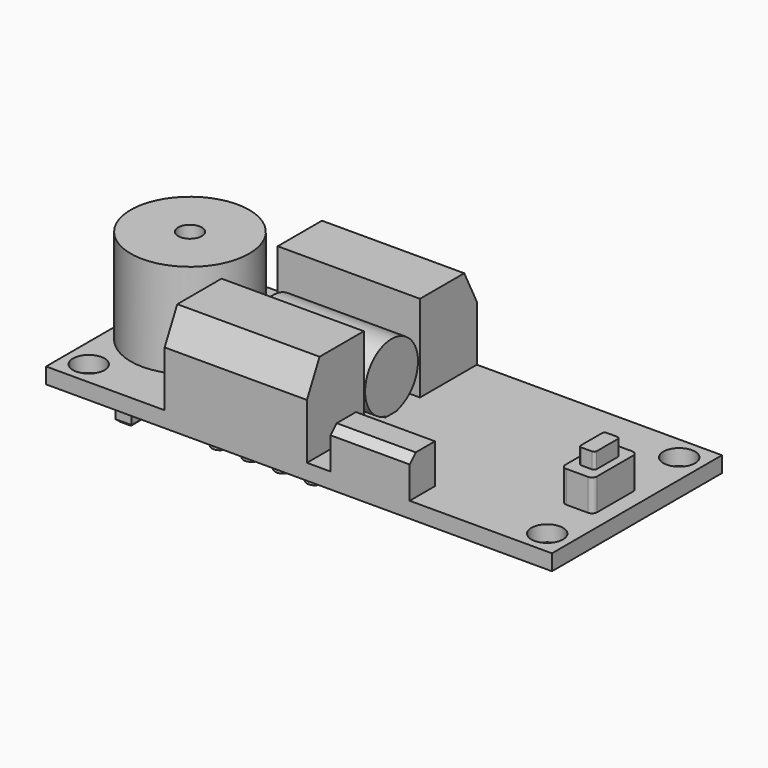
from build123d import *

# Parameters (mm, degrees)
F0_W      = 50.8
F0_H      = 21.336
F1_DEPTH  = 1.5875
F2_R      = 1.5875
F3_DEPTH  = 3.175
F5_DEPTH  = 2.38125
F6_W      = 1.5875
F6_H      = 2.38125
F6_W_2    = 5.55625
F6_H_2    = 3.96875
F6_W_3    = 2.38125
F6_H_3    = 3.175
F6_W_4    = 6.35
F6_H_4    = 4.7625
F7_DEPTH  = 1.5875
F8_SIZE   = 0.254
F9_W      = 5.55625
F9_H      = 7.14375
F10_DEPTH = 2.38125
F11_SIZE  = 0.762
F12_SIZE  = 0.254
F13_R     = 5.953125
F14_DEPTH = 9.525
F15_R     = 1.190625
F16_DEPTH = 3.175
F17_W     = 14.2875
F17_H     = 7.14375
F18_DEPTH = 8.73125
F20_DEPTH = 15.24
F22_DEPTH = 11.90625
F23_W     = 3.175
F23_H     = 5.55625
F24_DEPTH = 3.175
F25_W     = 1.5875
F25_H     = 3.175
F26_DEPTH = 1.5875
F27_R     = 0.254
F28_R     = 0.508
F29_W     = 7.9375
F29_H     = 3.175
F30_DEPTH = 3.96875
F31_SIZE  = 0.762


# Not quite as in the source:
# - a length typed as a fraction of an inch, garbled in the dataset ("3 / 203.2 mm" for 3/8 in), is restored


with BuildPart() as f1:
    # F0 (on Top) → F1 (new body)
    with BuildSketch(Plane.XY):
        with Locations((2.7589667588, 1.2681204271)):
            Rectangle(F0_W, F0_H)
    extrude(amount=F1_DEPTH)

    # F2 (on face) → F3 (cut)
    with BuildSketch(Plane.XY.offset(1.5875)):
        with Locations((25.7777167588, -7.0186295729)):
            Circle(F2_R)
        with Locations((25.7777167588, 9.5548704271)):
            Circle(F2_R)
        with Locations((-20.2597832412, 9.5548704271)):
            Circle(F2_R)
        with Locations((-20.2597832412, -7.0186295729)):
            Circle(F2_R)
    extrude(amount=-F3_DEPTH, mode=Mode.SUBTRACT)

    # F4 (on face) → F5 (join)
    with BuildSketch(Plane(origin=(0, 0, 0), x_dir=(1, 0, 0), z_dir=(0, 0, -1))):
        with BuildLine():
            ThreePointArc((-5.1785332412, 6.2248795729), (-5.9722832412, 5.4311295706), (-5.1785332365, 4.6373795729))
            ThreePointArc((-5.1785332365, 4.6373795729), (-4.6172672319, 4.869863567), (-4.3847832412, 5.4311295729))
            ThreePointArc((-4.3847832412, 5.4311295729), (-4.6172672336, 5.9923955805), (-5.1785332412, 6.2248795729))
        make_face()
        with BuildLine():
            ThreePointArc((-2.0035332412, 6.2248795729), (-2.7972832412, 5.4311295729), (-2.0035332412, 4.6373795729))
            ThreePointArc((-2.0035332412, 4.6373795729), (-1.4422672336, 4.8698635653), (-1.2097832412, 5.4311295729))
            ThreePointArc((-1.2097832412, 5.4311295729), (-1.4422672336, 5.9923955805), (-2.0035332412, 6.2248795729))
        make_face()
        with BuildLine():
            ThreePointArc((1.1714667642, 6.2248795729), (0.3777167588, 5.4311295756), (1.1714667588, 4.6373795729))
            ThreePointArc((1.1714667588, 4.6373795729), (1.7327327664, 4.8698635653), (1.9652167588, 5.4311295729))
            ThreePointArc((1.9652167588, 5.4311295729), (1.7327327683, 5.9923955786), (1.1714667642, 6.2248795729))
        make_face()
        with BuildLine():
            ThreePointArc((-7.5597832412, -7.1736204271), (-7.7922672336, -6.6123544195), (-8.3535332412, -6.3798704271))
            ThreePointArc((-8.3535332412, -6.3798704271), (-9.1472832412, -7.1736204294), (-8.3535332365, -7.9673704271))
            ThreePointArc((-8.3535332365, -7.9673704271), (-7.7922672319, -7.734886433), (-7.5597832412, -7.1736204271))
        make_face()
        with BuildLine():
            ThreePointArc((-4.3085832412, -7.1736204271), (-4.5410672336, -6.6123544195), (-5.1023332412, -6.3798704271))
            ThreePointArc((-5.1023332412, -6.3798704271), (-5.8960832412, -7.1736204294), (-5.1023332365, -7.9673704271))
            ThreePointArc((-5.1023332365, -7.9673704271), (-4.5410672319, -7.734886433), (-4.3085832412, -7.1736204271))
        make_face()
        with BuildLine():
            ThreePointArc((-1.0573832412, -7.1736204271), (-1.2898672336, -6.6123544195), (-1.8511332412, -6.3798704271))
            ThreePointArc((-1.8511332412, -6.3798704271), (-2.6448832412, -7.173620426), (-1.8511332433, -7.9673704271))
            ThreePointArc((-1.8511332433, -7.9673704271), (-1.2898672344, -7.7348864354), (-1.0573832412, -7.1736204271))
        make_face()
        with BuildLine():
            ThreePointArc((2.1938167588, -7.1736204271), (1.9613327682, -6.6123544213), (1.4000667639, -6.3798704271))
            ThreePointArc((1.4000667639, -6.3798704271), (0.6063167588, -7.1736204215), (1.4000667527, -7.9673704271))
            ThreePointArc((1.4000667527, -7.9673704271), (1.9613327642, -7.7348864368), (2.1938167588, -7.1736204271))
        make_face()
        with BuildLine():
            ThreePointArc((-8.3535332412, 6.2248795729), (-9.1472832412, 5.4311295729), (-8.3535332412, 4.6373795729))
            ThreePointArc((-8.3535332412, 4.6373795729), (-7.7922672336, 4.8698635653), (-7.5597832412, 5.4311295729))
            ThreePointArc((-7.5597832412, 5.4311295729), (-7.7922672336, 5.9923955805), (-8.3535332412, 6.2248795729))
        make_face()
    extrude(amount=F5_DEPTH)

    # F6 (on face) → F7 (join)
    with BuildSketch(Plane(origin=(0, 0, 0), x_dir=(1, 0, 0), z_dir=(0, 0, -1))):
        with Locations((-15.4972832412, 7.4155045729)):
            Rectangle(F6_W, F6_H)
        with Locations((-15.4972832412, 4.2405045729)):
            Rectangle(F6_W, F6_H)
        with Locations((-13.9097832412, -8.3642454271)):
            Rectangle(F6_W, F6_H)
        with Locations((-6.3691582412, 1.0655045729)):
            Rectangle(F6_W_2, F6_H_2)
        with Locations((0.7745917588, -0.1251204271)):
            Rectangle(F6_W_3, F6_H_3)
        with Locations((18.6339667588, 1.4623795729)):
            Rectangle(F6_W_4, F6_H_4)
        with Locations((18.2370917588, -4.7923704271)):
            Rectangle(F6_W_3, F6_H_4)
    extrude(amount=F7_DEPTH)

    # F8
    f8_edges = [f1.edges().sort_by_distance(p)[0] for p in [
        (-13.909783, 9.55487, -1.5875),
        (-13.116033, 8.364245, -1.5875),
        (-13.909783, 7.17362, -1.5875),
        (-14.703533, 8.364245, -1.5875),
        (-15.497283, -5.43113, -1.5875),
        (-16.291033, -4.240505, -1.5875),
        (-15.497283, -3.04988, -1.5875),
        (-14.703533, -4.240505, -1.5875),
        (-15.497283, -8.60613, -1.5875),
        (-16.291033, -7.415505, -1.5875),
        (-15.497283, -6.22488, -1.5875),
        (-14.703533, -7.415505, -1.5875),
        (-3.591033, -1.065505, -1.5875),
        (-6.369158, -3.04988, -1.5875),
        (-9.147283, -1.065505, -1.5875),
        (-6.369158, 0.91887, -1.5875),
        (0.774592, 1.71262, -1.5875),
        (1.965217, 0.12512, -1.5875),
        (0.774592, -1.46238, -1.5875),
        (-0.416033, 0.12512, -1.5875),
        (18.633967, 0.91887, -1.5875),
        (21.808967, -1.46238, -1.5875),
        (18.633967, -3.84363, -1.5875),
        (15.458967, -1.46238, -1.5875),
        (19.427717, 4.79237, -1.5875),
        (18.237092, 2.41112, -1.5875),
        (17.046467, 4.79237, -1.5875),
        (18.237092, 7.17362, -1.5875),
    ]]
    chamfer(f8_edges, length=F8_SIZE)

    # F9 (on face) → F10 (join)
    with BuildSketch(Plane(origin=(0, 0, 0), x_dir=(1, 0, 0), z_dir=(0, 0, -1))):
        with Locations((7.9183417588, -2.1094954271)):
            Rectangle(F9_W, F9_H)
    extrude(amount=F10_DEPTH)

    # F11
    f11_edges = [f1.edges().sort_by_distance(p)[0] for p in [
        (10.696467, 2.109495, -2.38125),
        (5.140217, 2.109495, -2.38125),
    ]]
    chamfer(f11_edges, length=F11_SIZE)

    # F12
    f12_edges = [f1.edges().sort_by_distance(p)[0] for p in [
        (7.918342, -1.46238, -2.38125),
        (7.918342, 5.68137, -2.38125),
    ]]
    chamfer(f12_edges, length=F12_SIZE)

    # F13 (on face) → F14 (join)
    with BuildSketch(Plane.XY.offset(1.5875)):
        with Locations((-16.6879082412, 1.2204954271)):
            Circle(F13_R)
    extrude(amount=F14_DEPTH)

    # F15 (on face) → F16 (cut)
    with BuildSketch(Plane.XY.offset(11.1125)):
        with Locations((-16.6879082412, 1.2204954271)):
            Circle(F15_R)
    extrude(amount=-F16_DEPTH, mode=Mode.SUBTRACT)

    # F17 (on face) → F18 (join)
    with BuildSketch(Plane.XY.offset(1.5875)):
        with Locations((-3.5910332412, 8.3642454271)):
            Rectangle(F17_W, F17_H)
        with Locations((-3.5910332412, -5.8280045729)):
            Rectangle(F17_W, F17_H)
    extrude(amount=F18_DEPTH)

    # F19 (on face) → F20 (cut)
    with BuildSketch(Plane.YZ.offset(3.5527167588)):
        Polygon((-12.6245096326, 12.3970924459), (-9.3998795729, 7.14375), (-7.8123795729, 10.31875), (-6.8544447422, 13.4305364035), align=None)
        Polygon((11.640425374, 13.160722746), (10.3486204271, 10.31875), (11.9361204271, 7.14375), (15.5531742786, 9.6412404954), (16.3770463069, 13.6774447247), align=None)
    extrude(amount=-F20_DEPTH, mode=Mode.SUBTRACT)

    # F21 (on face) → F22 (join)
    with BuildSketch(Plane.YZ.offset(3.5527167588)):
        with BuildLine():
            ThreePointArc((1.9973354259, 1.6797255876), (3.8268101171, 2.8522266244), (4.5383704271, 4.905375))
            ThreePointArc((4.5383704271, 4.905375), (-0.8326529485, 7.51168969), (0.4436554283, 1.6797255876))
            Line((0.4436554283, 1.6797255876), (1.9973354259, 1.6797255876))
        make_face()
        with BuildLine():
            Line((1.9973354259, 1.6797255876), (0.4436554283, 1.6797255876))
            ThreePointArc((0.4436554283, 1.6797255876), (1.2204954271, 1.5875), (1.9973354259, 1.6797255876))
        make_face()
        with BuildLine():
            ThreePointArc((1.9973354259, 1.6797255876), (1.2204954271, 1.5875), (0.4436554283, 1.6797255876))
            Line((0.4436554283, 1.6797255876), (0.4436554283, 1.5345554566))
            Line((0.4436554283, 1.5345554566), (1.9973354259, 1.5345554566))
            Line((1.9973354259, 1.5345554566), (1.9973354259, 1.6797255876))
        make_face()
    extrude(amount=-F22_DEPTH)

    # F23 (on face) → F24 (join)
    with BuildSketch(Plane.XY.offset(1.5875)):
        with Locations((24.9839667588, 0.5219954271)):
            Rectangle(F23_W, F23_H)
    extrude(amount=F24_DEPTH)

    # F25 (on face) → F26 (join)
    with BuildSketch(Plane.XY.offset(4.7625)):
        with Locations((24.9839667588, 0.5219954271)):
            Rectangle(F25_W, F25_H)
    extrude(amount=F26_DEPTH)

    # F27
    f27_edges = [f1.edges().sort_by_distance(p)[0] for p in [
        (25.777717, -1.065505, 5.55625),
        (24.190217, -1.065505, 5.55625),
        (24.190217, 2.109495, 5.55625),
        (25.777717, 2.109495, 5.55625),
    ]]
    fillet(f27_edges, radius=F27_R)

    # F28
    f28_edges = [f1.edges().sort_by_distance(p)[0] for p in [
        (26.571467, 3.30012, 3.175),
        (23.396467, 3.30012, 3.175),
        (26.571467, -2.25613, 3.175),
        (23.396467, -2.25613, 3.175),
    ]]
    fillet(f28_edges, radius=F28_R)

    # F29 (on face) → F30 (join)
    with BuildSketch(Plane.XY.offset(1.5875)):
        with Locations((9.9027167588, -7.8123795729)):
            Rectangle(F29_W, F29_H)
    extrude(amount=F30_DEPTH)

    # F31
    f31_edges = [f1.edges().sort_by_distance(p)[0] for p in [
        (9.902717, -9.39988, 5.55625),
    ]]
    chamfer(f31_edges, length=F31_SIZE)


solid = f1.part
